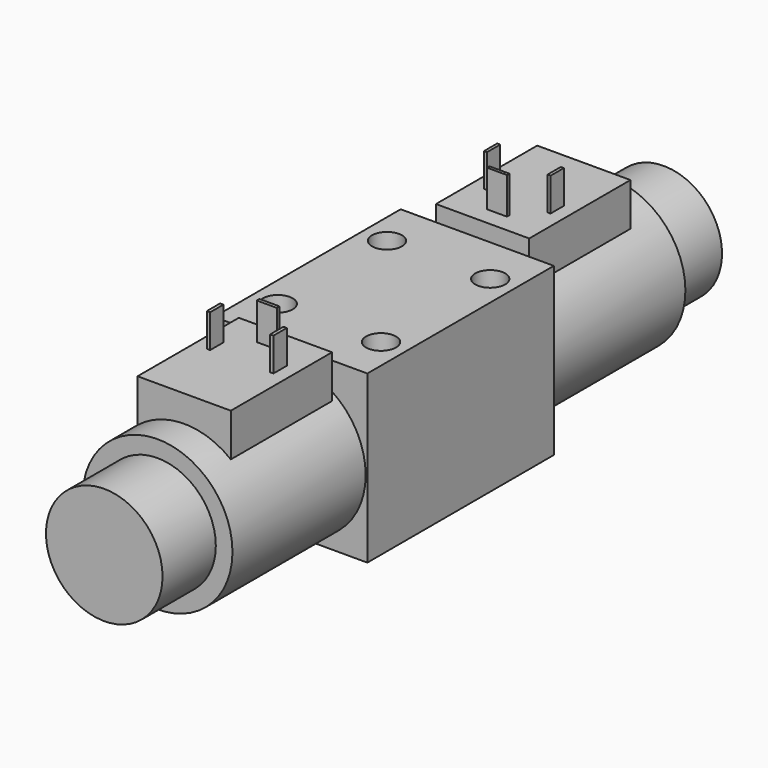
from build123d import *

# Parameters (mm, degrees)
F0_R      = 22.5
F1_DEPTH  = 50
F2_W      = 46
F2_H      = 50
F2_R      = 22.5
F3_DEPTH  = 70
F4_R      = 22.5
F5_DEPTH  = 50
F6_R      = 17.5
F7_DEPTH  = 20
F8_R      = 17.5
F9_DEPTH  = 20
F10_W     = 28
F10_H     = 38
F11_DEPTH = 30.5
F12_W     = 28
F12_H     = 38
F13_DEPTH = 30.5
F15_R     = 2.5
F16_DEPTH = 50
F14_R     = 4.5
F17_DEPTH = 11
F18_W     = 6
F18_H     = 0.9020372182
F19_DEPTH = 11
F20_W     = 6
F20_H     = 1
F21_DEPTH = 11
F20_W_2   = 1
F20_H_2   = 5
F22_DEPTH = 10
F18_W_2   = 0.9020372182
F18_H_2   = 5
F23_DEPTH = 10


# Not quite as in the source:
# - a feature names something its author has since deleted; it is built from what else it names


with BuildPart() as f1:
    # F0 (on Front) → F1 (new body)
    with BuildSketch(Plane.XZ):
        Circle(F0_R)
    extrude(amount=F1_DEPTH)

    # F2 (on face) → F3 (join)
    with BuildSketch(Plane.XZ.offset(50)):
        with Locations((0, 2)):
            Rectangle(F2_W, F2_H)
        Circle(F2_R, mode=Mode.SUBTRACT)
        Circle(F2_R)
    extrude(amount=F3_DEPTH)

    # F4 (on face) → F5 (join)
    with BuildSketch(Plane.XZ.offset(120)):
        Circle(F4_R)
    extrude(amount=F5_DEPTH)

    # F6 (on face) → F7 (join)
    with BuildSketch(Plane.XZ.offset(170)):
        Circle(F6_R)
    extrude(amount=F7_DEPTH)

    # F8 (on face) → F9 (join)
    with BuildSketch(Plane(origin=(0, 0, 0), x_dir=(-1, 0, 0), z_dir=(0, 1, 0))):
        Circle(F8_R)
    extrude(amount=F9_DEPTH)

    # F10 (on Top) → F11 (join)
    with BuildSketch(Plane.XY):
        with Locations((0, -29)):
            Rectangle(F10_W, F10_H)
    extrude(amount=F11_DEPTH)

    # F12 (on Top) → F13 (join)
    with BuildSketch(Plane.XY):
        with Locations((0, -141)):
            Rectangle(F12_W, F12_H)
    extrude(amount=F13_DEPTH)

    # F15 (on face) → F16 (cut)
    with BuildSketch(Plane.XY.offset(27)):
        with Locations((-15.5, -64.5)):
            Circle(F15_R)
        with Locations((-15.5, -105.5)):
            Circle(F15_R)
        with Locations((15.5, -105.5)):
            Circle(F15_R)
        with Locations((15.5, -64.5)):
            Circle(F15_R)
    extrude(amount=-F16_DEPTH, mode=Mode.SUBTRACT)

    # F14 (on face) → F17 (cut)
    with BuildSketch(Plane.XY.offset(27)):
        with Locations((-15.5, -64.5)):
            Circle(F14_R)
        with Locations((15.5, -64.5)):
            Circle(F14_R)
        with Locations((15.5, -105.5)):
            Circle(F14_R)
        with Locations((-15.5, -105.5)):
            Circle(F14_R)
    extrude(amount=-F17_DEPTH, mode=Mode.SUBTRACT)

    # F18 (on face) → F19 (join)
    with BuildSketch(Plane.XY.offset(30.5)):
        with Locations((0, -42.164042592)):
            Rectangle(F18_W, F18_H)
    extrude(amount=F19_DEPTH)

    # F20 (on face) → F21 (join)
    with BuildSketch(Plane.XY.offset(30.5)):
        with Locations((0, -128.5)):
            Rectangle(F20_W, F20_H)
    extrude(amount=F21_DEPTH)

    # F20 (on face) → F22 (join)
    with BuildSketch(Plane.XY.offset(30.5)):
        with Locations((9.5, -136.5)):
            Rectangle(F20_W_2, F20_H_2)
        with Locations((0, -128.5)):
            Rectangle(F20_W, F20_H)
        with Locations((-9.5, -136.5)):
            Rectangle(F20_W_2, F20_H_2)
    extrude(amount=F22_DEPTH)

    # F18 (on face) → F23 (join)
    with BuildSketch(Plane.XY.offset(30.5)):
        with Locations((-9.5489813909, -32.5)):
            Rectangle(F18_W_2, F18_H_2)
        with Locations((9.5489813909, -32.5)):
            Rectangle(F18_W_2, F18_H_2)
        with Locations((0, -42.164042592)):
            Rectangle(F18_W, F18_H)
    extrude(amount=F23_DEPTH)


solid = f1.part
